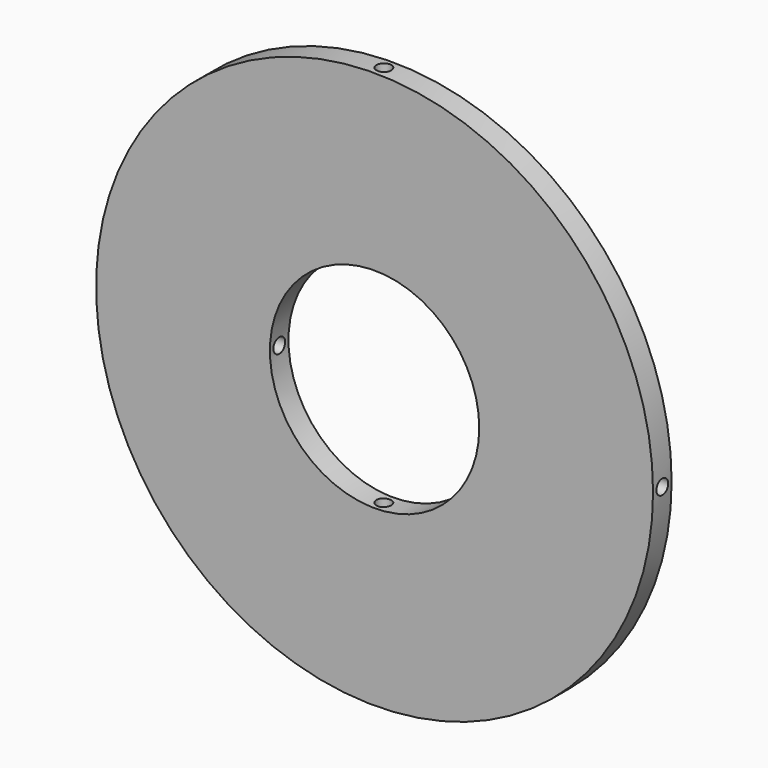
from build123d import *

# Parameters (mm, degrees)
F0_R     = 76.2
F0_R_2   = 28.6385
F1_DEPTH = 6.35
F4_D     = 4.0386
F7_D     = 4.0386


# Not quite as in the source:
# - a feature names something its author has since deleted; it is built from what else it names


with BuildPart() as f1:
    # F0 (on Front) → F1 (new body)
    with BuildSketch(Plane.XZ):
        Circle(F0_R)
        Circle(F0_R_2, mode=Mode.SUBTRACT)
    extrude(amount=F1_DEPTH)

    # F4 (through all)
    with Locations(Plane.XY.offset(76.2)):
        with Locations((0, -3.175)):
            Hole(F4_D / 2)

    # F7 (through all)
    with Locations(Plane.YZ.offset(76.2)):
        with Locations((-3.175, 0)):
            Hole(F7_D / 2)


solid = f1.part
